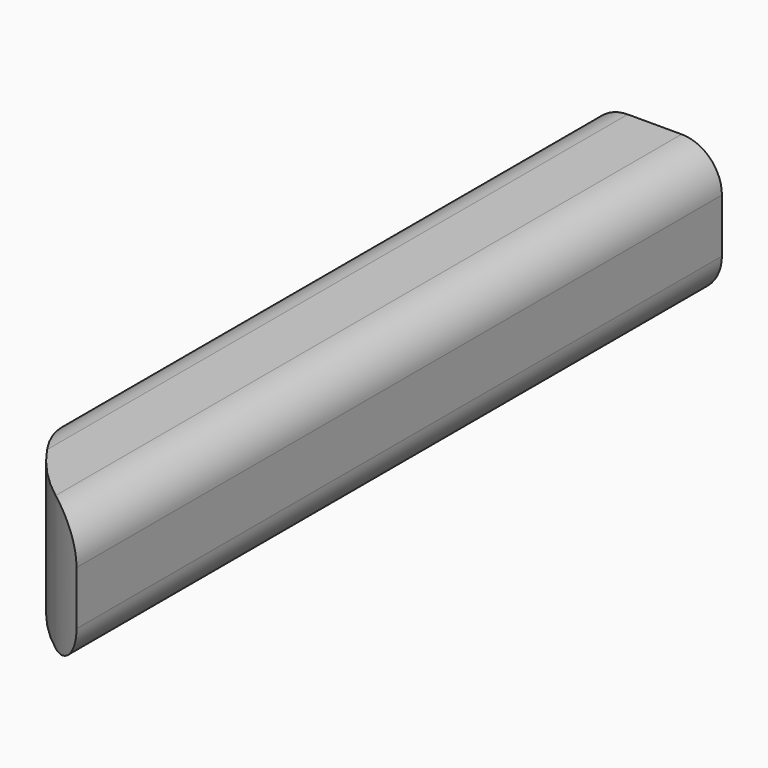
from build123d import *

# Parameters (mm, degrees)
F0_W        = 25.4
F0_H        = 25.4
F1_DEPTH    = 152.4
F2_R        = 7.62
F3_T1_DEPTH = 190.5
F4_R        = 7.62
F5_T1_DEPTH = 190.5
F6_T1_DEPTH = 210.9646314207


# Not quite as in the source:
# - a fillet or chamfer that OpenCascade refuses, or shapes differently, is made with other operations: its cross-section is extruded or revolved along the edge and cut away or added


with BuildPart() as f1:
    # F0 (on Front) → F1 (new body)
    with BuildSketch(Plane.XZ):
        with Locations((12.7, -12.7)):
            Rectangle(F0_W, F0_H)
    extrude(amount=-F1_DEPTH)

    # F2
    f2_edges = [f1.edges().sort_by_distance(p)[0] for p in [
        (25.4, 76.2, 0),
    ]]
    fillet(f2_edges, radius=F2_R)

    # F3: fillet of radius 7.62 on 1 edges, made by hand

    # F3_s2 → F3_t1 (cut)
    with BuildSketch(Plane.XZ.offset(-171.45)):
        with BuildLine():
            ThreePointArc((7.62, 0), (2.2318463274, -2.2318463274), (0, -7.62))
            Line((0, -7.62), (0, 0))
            Line((0, 0), (7.62, 0))
        make_face()
    extrude(amount=F3_T1_DEPTH, mode=Mode.SUBTRACT)

    # F4
    f4_edges = [f1.edges().sort_by_distance(p)[0] for p in [
        (25.4, 76.2, -25.4),
    ]]
    fillet(f4_edges, radius=F4_R)

    # F5: fillet of radius 7.62 on 1 edges, made by hand

    # F5_s2 → F5_t1 (cut)
    with BuildSketch(Plane.XZ.offset(-171.45)):
        with BuildLine():
            ThreePointArc((7.62, -25.4), (2.2318463274, -23.1681536726), (0, -17.78))
            Line((0, -17.78), (0, -25.4))
            Line((0, -25.4), (7.62, -25.4))
        make_face()
    extrude(amount=F5_T1_DEPTH, mode=Mode.SUBTRACT)

    # F6: fillet of radius 44.45 on 1 edges, made by hand

    # F6_s2 → F6_t1 (cut)
    with BuildSketch(Plane.XY.offset(-118.1823157103)):
        with BuildLine():
            ThreePointArc((25.4, 0), (6.8828933773, 16.4014018781), (0, 40.1609262841))
            Line((0, 40.1609262841), (0, 0))
            Line((0, 0), (25.4, 0))
        make_face()
    extrude(amount=F6_T1_DEPTH, mode=Mode.SUBTRACT)


solid = f1.part
